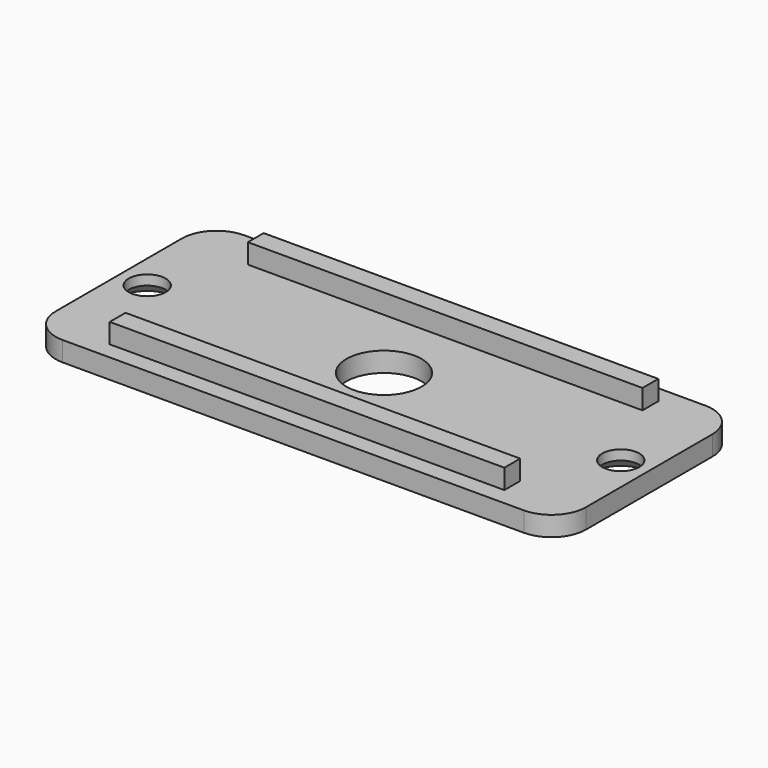
from build123d import *

# Parameters (mm, degrees)
F1_DEPTH = 2
F2_R     = 1.875
F3_DEPTH = 2.001
F4_SIZE  = 0.99999
F5_W     = 40
F5_H     = 2
F6_DEPTH = 2
F7_R     = 3.81
F8_DEPTH = 2.001


# Not quite as in the source:
# - a fillet or chamfer is up to 0.001 mm smaller than in the source, because OpenCascade refuses the exact size


with BuildPart() as f1:
    # F0 (on Top) → F1 (new body)
    with BuildSketch(Plane.XY):
        with BuildLine():
            ThreePointArc((26.875, 8), (25.8498737342, 10.4748737342), (23.375, 11.5))
            Line((23.375, 11.5), (-23.375, 11.5))
            ThreePointArc((-23.375, 11.5), (-25.8498737342, 10.4748737342), (-26.875, 8))
            Line((-26.875, 8), (-26.875, -8))
            ThreePointArc((-26.875, -8), (-25.8498737342, -10.4748737342), (-23.375, -11.5))
            Line((-23.375, -11.5), (23.375, -11.5))
            ThreePointArc((23.375, -11.5), (25.8498737342, -10.4748737342), (26.875, -8))
            Line((26.875, -8), (26.875, 8))
        make_face()
    extrude(amount=F1_DEPTH)

    # F2 (on face) → F3 (cut, through all)
    with BuildSketch(Plane.XY.offset(2)):
        with Locations((-24, 0)):
            Circle(F2_R)
        with Locations((24, 0)):
            Circle(F2_R)
    extrude(amount=-F3_DEPTH, mode=Mode.SUBTRACT)

    # F4 (size 1 in the source; OpenCascade refuses exactly that, so slightly less here)
    f4_edges = [f1.edges().sort_by_distance(p)[0] for p in [
        (-25.875, 0, 0),
        (22.125, 0, 0),
    ]]
    chamfer(f4_edges, length=F4_SIZE)

    # F5 (on face) → F6 (join)
    with BuildSketch(Plane.XY.offset(2)):
        with Locations((0, 8.75)):
            Rectangle(F5_W, F5_H)
        with Locations((0, -8.75)):
            Rectangle(F5_W, F5_H)
    extrude(amount=F6_DEPTH)

    # F7 (on face) → F8 (cut, through all)
    with BuildSketch(Plane.XY.offset(2)):
        Circle(F7_R)
    extrude(amount=-F8_DEPTH, mode=Mode.SUBTRACT)


solid = f1.part
